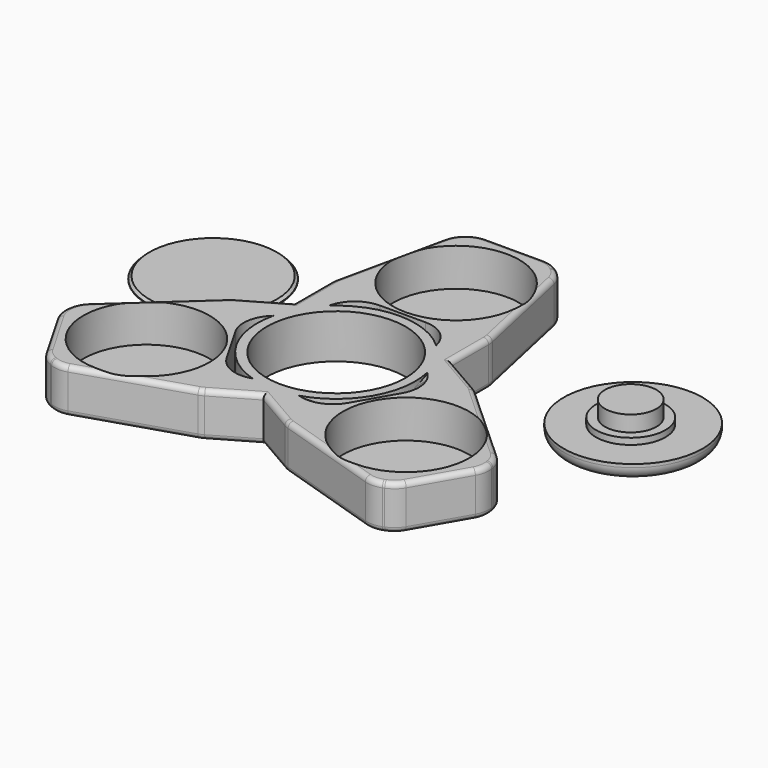
from build123d import *

# Parameters (mm, degrees)
F0_R         = 11
F1_DEPTH     = 7
F0_R_2       = 10
F2_DEPTH     = 7
F3_DEPTH     = 1
F4_SIZE      = 2
F5_R         = 4
F6_T3_DEPTH  = 17.2209539542
F6_T6_ANGLE  = 38.8320169601
F6_T9_ANGLE  = 38.8320169601
F6_T12_DEPTH = 9.1802464008
F6_T15_DEPTH = 0.2962051646
F6_T18_ANGLE = 38.8319208499
F6_T21_ANGLE = 38.8319208499
F6_T24_DEPTH = 17.2206278221
F6_T27_ANGLE = 12.3359660798
F6_T30_ANGLE = 38.8320169601
F6_T33_ANGLE = 38.8320169601
F6_T36_DEPTH = 17.2209539542
F6_T39_DEPTH = 9.1802464008
F6_T42_ANGLE = 38.8319208499
F6_T45_ANGLE = 38.8319208499
F6_T48_DEPTH = 17.2206278221
F6_T51_DEPTH = 0.2962051646
F6_T54_DEPTH = 0.2961934139
F6_T57_ANGLE = 12.3361583003
F6_T60_ANGLE = 12.3359660798
F6_T63_DEPTH = 0.2961934139
F6_T66_ANGLE = 12.3361583003
F6_T69_DEPTH = 14.5444922906
F6_S70_R     = 12.5
F6_T71_DEPTH = 9
F6_T74_DEPTH = 14.5441683265
F6_S75_R     = 12.5
F6_T76_DEPTH = 9
F6_T79_DEPTH = 14.5444922906
F6_S80_R     = 12.5
F6_T81_DEPTH = 9
F6_T84_DEPTH = 14.5441683265
F6_S85_R     = 12.5
F6_T86_DEPTH = 9
F7_T1_DEPTH  = 7
F8_COUNT     = 3
F9_R         = 10.5
F10_DEPTH    = 0.5
F11_SIZE     = 0.4
F12_R        = 11
F12_R_2      = 5.5
F13_DEPTH    = 2.5
F12_R_3      = 4.075
F14_DEPTH    = 3.5
F15_DEPTH    = 6
F16_R        = 2


# Not quite as in the source:
# - a fillet or chamfer that OpenCascade refuses, or shapes differently, is made with other operations: its cross-section is extruded or revolved along the edge and cut away or added


with BuildPart() as f1:
    # F0 (on Top) → F1 (new body)
    with BuildSketch(Plane.XY):
        with BuildLine():
            ThreePointArc((-12.5, 0), (0, -12.5), (12.5, 0))
            ThreePointArc((12.5, 0), (11.4564392374, 5), (8.5, 9.1651513899))
            ThreePointArc((8.5, 9.1651513899), (0, 12.5), (-8.5, 9.1651513899))
            ThreePointArc((-8.5, 9.1651513899), (-11.4564392374, 5), (-12.5, 0))
        make_face()
        Circle(F0_R, mode=Mode.SUBTRACT)
    extrude(amount=F1_DEPTH)

    # F0 (on Top) → F2 (join)
    with BuildSketch(Plane.XY):
        with BuildLine():
            ThreePointArc((8.5, 9.1651513899), (11.4564392374, 5), (12.5, 0))
            Line((12.5, 0), (12.5, 14.9764459367))
            Line((12.5, 14.9764459367), (8, 35.553243875))
            Line((8, 35.553243875), (0, 35.553243875))
            Line((0, 35.553243875), (-8, 35.553243875))
            Line((-8, 35.553243875), (-12.5, 14.9767766889))
            Line((-12.5, 14.9767766889), (-12.5, 0))
            ThreePointArc((-12.5, 0), (-11.4564392374, 5), (-8.5, 9.1651513899))
            Line((-8.5, 9.1651513899), (-8.5, 13.1651513899))
            Line((-8.5, 13.1651513899), (8.5, 13.1651513899))
            Line((8.5, 13.1651513899), (8.5, 9.1651513899))
        make_face()
        with Locations((0, 23.7397756428)):
            Circle(F0_R_2, mode=Mode.SUBTRACT)
    extrude(amount=F2_DEPTH)

    # F0 (on Top) → F3 (join)
    with BuildSketch(Plane.XY):
        with Locations((0, 23.7397756428)):
            Circle(F0_R_2)
    extrude(amount=F3_DEPTH)

    # F4
    f4_edges = [f1.edges().sort_by_distance(p)[0] for p in [
        (8, 35.553244, 3.5),
        (-8, 35.553244, 3.5),
    ]]
    chamfer(f4_edges, length=F4_SIZE)

    # F5
    f5_edges = [f1.edges().sort_by_distance(p)[0] for p in [
        (8.427287, 33.599421, 3.5),
        (6, 35.553244, 3.5),
        (-6, 35.553244, 3.5),
        (-8.427294, 33.599422, 3.5),
        (-12.5, 14.976777, 3.5),
        (12.5, 14.976446, 3.5),
    ]]
    fillet(f5_edges, radius=F5_R)

    # F6: fillet of radius 0.8 on 22 edges, made by hand


with BuildPart() as f6_tool1:
    # F6_s2 → F6_t3 (new body)
    with BuildSketch(Plane(origin=(-2.647556956, 12.1062765587, 0), x_dir=(0, 0, 1), z_dir=(-0.2136436617, 0.9769116571, 0))):
        with BuildLine():
            ThreePointArc((7, 14.6110184628), (6.7656854249, 15.1767038878), (6.2, 15.4110184628))
            Line((6.2, 15.4110184628), (7, 15.4110184628))
            Line((7, 15.4110184628), (7, 14.6110184628))
        make_face()
    extrude(amount=F6_T3_DEPTH)


with BuildPart() as f6_tool4:
    # F6_s5 → F6_t6 (revolve)
    with BuildSketch(Plane(origin=(-6.3267046163, 28.9296272233, 0), x_dir=(0, 0, 1), z_dir=(0.2136436617, -0.9769116571, 0))):
        with BuildLine():
            ThreePointArc((7, -14.6110184628), (6.7656854249, -15.1767038878), (6.2, -15.4110184628))
            Line((6.2, -15.4110184628), (7, -15.4110184628))
            Line((7, -15.4110184628), (7, -14.6110184628))
        make_face()
    revolve(axis=Axis((4.8208523397, 31.3675189911, 7), (0, 0, 1)), revolution_arc=F6_T6_ANGLE)


with BuildPart() as f6_tool7:
    # F6_s8 → F6_t9 (revolve)
    with BuildSketch(Plane(origin=(-12.6269800609, 10.163975148, 0), x_dir=(0, 0, 1), z_dir=(0.7789876962, -0.6270392086, 0))):
        with BuildLine():
            ThreePointArc((7, -30.6577747906), (6.7656854249, -31.2234602155), (6.2, -31.4577747906))
            Line((6.2, -31.4577747906), (7, -31.4577747906))
            Line((7, -31.4577747906), (7, -30.6577747906))
        make_face()
    revolve(axis=Axis((4.5901213146, 31.553243875, 7), (0, 0, 1)), revolution_arc=F6_T9_ANGLE)


with BuildPart() as f6_tool10:
    # F6_s11 → F6_t12 (new body)
    with BuildSketch(Plane.YZ.offset(-4.5901250862)):
        with BuildLine():
            ThreePointArc((34.753243875, 7), (35.3189293, 6.7656854249), (35.553243875, 6.2))
            Line((35.553243875, 6.2), (35.553243875, 7))
            Line((35.553243875, 7), (34.753243875, 7))
        make_face()
    extrude(amount=F6_T12_DEPTH)


with BuildPart() as f6_tool13:
    # F6_s14 → F6_t15 (new body)
    with BuildSketch(Plane(origin=(12.6269589424, 10.1639232441, 0), x_dir=(0, 0, 1), z_dir=(-0.778988748, -0.6270379019, 0))):
        with BuildLine():
            ThreePointArc((7, 30.6578043459), (6.7656854249, 31.2234897709), (6.2, 31.4578043459))
            Line((6.2, 31.4578043459), (7, 31.4578043459))
            Line((7, 31.4578043459), (7, 30.6578043459))
        make_face()
    extrude(amount=F6_T15_DEPTH)


with BuildPart() as f6_tool16:
    # F6_s17 → F6_t18 (revolve)
    with BuildSketch(Plane.YZ.offset(-4.5901250862)):
        with BuildLine():
            ThreePointArc((34.753243875, 7), (35.3189293, 6.7656854249), (35.553243875, 6.2))
            Line((35.553243875, 6.2), (35.553243875, 7))
            Line((35.553243875, 7), (34.753243875, 7))
        make_face()
    revolve(axis=Axis((-4.5901250862, 31.553243875, 7), (0, 0, 1)), revolution_arc=F6_T18_ANGLE)


with BuildPart() as f6_tool19:
    # F6_s20 → F6_t21 (revolve)
    with BuildSketch(Plane(origin=(12.3962184521, 9.9781913792, 0), x_dir=(0, 0, 1), z_dir=(0.778988748, 0.6270379019, 0))):
        with BuildLine():
            ThreePointArc((7, -30.6578043459), (6.7656854249, -31.2234897709), (6.2, -31.4578043459))
            Line((6.2, -31.4578043459), (7, -31.4578043459))
            Line((7, -31.4578043459), (7, -30.6578043459))
        make_face()
    revolve(axis=Axis((-4.8208655765, 31.3675120101, 7), (0, 0, 1)), revolution_arc=F6_T21_ANGLE)


with BuildPart() as f6_tool22:
    # F6_s23 → F6_t24 (new body)
    with BuildSketch(Plane(origin=(6.3267914314, 28.9295591739, 0), x_dir=(0, 0, 1), z_dir=(-0.2136469391, -0.9769109404, 0))):
        with BuildLine():
            ThreePointArc((7, 14.6111292517), (6.7656854249, 15.1768146767), (6.2, 15.4111292517))
            Line((6.2, 15.4111292517), (7, 15.4111292517))
            Line((7, 15.4111292517), (7, 14.6111292517))
        make_face()
    extrude(amount=F6_T24_DEPTH)


with BuildPart() as f6_tool25:
    # F6_s26 → F6_t27 (revolve)
    with BuildSketch(Plane(origin=(-2.647556956, 12.1062765587, 0), x_dir=(0, 0, 1), z_dir=(-0.2136436617, 0.9769116571, 0))):
        with BuildLine():
            ThreePointArc((7, 14.6110184628), (6.7656854249, 15.1767038878), (6.2, 15.4110184628))
            Line((6.2, 15.4110184628), (7, 15.4110184628))
            Line((7, 15.4110184628), (7, 14.6110184628))
        make_face()
    revolve(axis=Axis((8.5, 14.5441683265, 7), (0, 0, -1)), revolution_arc=F6_T27_ANGLE)


with BuildPart() as f6_tool28:
    # F6_s29 → F6_t30 (revolve)
    with BuildSketch(Plane(origin=(-12.6269800609, 10.163975148, 0), x_dir=(0, 0, 1), z_dir=(0.7789876962, -0.6270392086, 0))):
        with BuildLine():
            ThreePointArc((0.8, -31.4577747906), (0.2343145751, -31.2234602155), (0, -30.6577747906))
            Line((0, -30.6577747906), (0, -31.4577747906))
            Line((0, -31.4577747906), (0.8, -31.4577747906))
        make_face()
    revolve(axis=Axis((4.5901213146, 31.553243875, 0), (0, 0, 1)), revolution_arc=F6_T30_ANGLE)


with BuildPart() as f6_tool31:
    # F6_s32 → F6_t33 (revolve)
    with BuildSketch(Plane(origin=(-6.3267046163, 28.9296272233, 0), x_dir=(0, 0, 1), z_dir=(0.2136436617, -0.9769116571, 0))):
        with BuildLine():
            ThreePointArc((0.8, -15.4110184628), (0.2343145751, -15.1767038878), (0, -14.6110184628))
            Line((0, -14.6110184628), (0, -15.4110184628))
            Line((0, -15.4110184628), (0.8, -15.4110184628))
        make_face()
    revolve(axis=Axis((4.8208523397, 31.3675189911, 0), (0, 0, 1)), revolution_arc=F6_T33_ANGLE)


with BuildPart() as f6_tool34:
    # F6_s35 → F6_t36 (new body)
    with BuildSketch(Plane(origin=(-2.647556956, 12.1062765587, 0), x_dir=(0, 0, 1), z_dir=(-0.2136436617, 0.9769116571, 0))):
        with BuildLine():
            ThreePointArc((0.8, 15.4110184628), (0.2343145751, 15.1767038878), (0, 14.6110184628))
            Line((0, 14.6110184628), (0, 15.4110184628))
            Line((0, 15.4110184628), (0.8, 15.4110184628))
        make_face()
    extrude(amount=F6_T36_DEPTH)


with BuildPart() as f6_tool37:
    # F6_s38 → F6_t39 (new body)
    with BuildSketch(Plane.YZ.offset(4.5901213146)):
        with BuildLine():
            ThreePointArc((35.553243875, 0.8), (35.3189293, 0.2343145751), (34.753243875, 0))
            Line((34.753243875, 0), (35.553243875, 0))
            Line((35.553243875, 0), (35.553243875, 0.8))
        make_face()
    extrude(amount=-F6_T39_DEPTH)


with BuildPart() as f6_tool40:
    # F6_s41 → F6_t42 (revolve)
    with BuildSketch(Plane.YZ.offset(-4.5901250862)):
        with BuildLine():
            ThreePointArc((35.553243875, 0.8), (35.3189293, 0.2343145751), (34.753243875, 0))
            Line((34.753243875, 0), (35.553243875, 0))
            Line((35.553243875, 0), (35.553243875, 0.8))
        make_face()
    revolve(axis=Axis((-4.5901250862, 31.553243875, 0), (0, 0, 1)), revolution_arc=F6_T42_ANGLE)


with BuildPart() as f6_tool43:
    # F6_s44 → F6_t45 (revolve)
    with BuildSketch(Plane(origin=(12.3962184521, 9.9781913792, 0), x_dir=(0, 0, 1), z_dir=(0.778988748, 0.6270379019, 0))):
        with BuildLine():
            ThreePointArc((0.8, -31.4578043459), (0.2343145751, -31.2234897709), (0, -30.6578043459))
            Line((0, -30.6578043459), (0, -31.4578043459))
            Line((0, -31.4578043459), (0.8, -31.4578043459))
        make_face()
    revolve(axis=Axis((-4.8208655765, 31.3675120101, 0), (0, 0, 1)), revolution_arc=F6_T45_ANGLE)


with BuildPart() as f6_tool46:
    # F6_s47 → F6_t48 (new body)
    with BuildSketch(Plane(origin=(6.3267914314, 28.9295591739, 0), x_dir=(0, 0, 1), z_dir=(-0.2136469391, -0.9769109404, 0))):
        with BuildLine():
            ThreePointArc((0.8, 15.4111292517), (0.2343145751, 15.1768146767), (0, 14.6111292517))
            Line((0, 14.6111292517), (0, 15.4111292517))
            Line((0, 15.4111292517), (0.8, 15.4111292517))
        make_face()
    extrude(amount=F6_T48_DEPTH)


with BuildPart() as f6_tool49:
    # F6_s50 → F6_t51 (new body)
    with BuildSketch(Plane(origin=(12.6269589424, 10.1639232441, 0), x_dir=(0, 0, 1), z_dir=(-0.778988748, -0.6270379019, 0))):
        with BuildLine():
            ThreePointArc((0.8, 31.4578043459), (0.2343145751, 31.2234897709), (0, 30.6578043459))
            Line((0, 30.6578043459), (0, 31.4578043459))
            Line((0, 31.4578043459), (0.8, 31.4578043459))
        make_face()
    extrude(amount=F6_T51_DEPTH)


with BuildPart() as f6_tool52:
    # F6_s53 → F6_t54 (new body)
    with BuildSketch(Plane(origin=(-12.3962490358, 9.9782502642, 0), x_dir=(0, 0, 1), z_dir=(-0.7789876962, 0.6270392086, 0))):
        with BuildLine():
            ThreePointArc((7, 30.6577747906), (6.7656854249, 31.2234602155), (6.2, 31.4577747906))
            Line((6.2, 31.4577747906), (7, 31.4577747906))
            Line((7, 31.4577747906), (7, 30.6577747906))
        make_face()
    extrude(amount=F6_T54_DEPTH)


with BuildPart() as f6_tool55:
    # F6_s56 → F6_t57 (revolve)
    with BuildSketch(Plane.XZ.offset(-14.5444922906)):
        with BuildLine():
            ThreePointArc((-11.7, 7), (-12.2656854249, 6.7656854249), (-12.5, 6.2))
            Line((-12.5, 6.2), (-12.5, 7))
            Line((-12.5, 7), (-11.7, 7))
        make_face()
    revolve(axis=Axis((-8.5, 14.5444922906, 7), (0, 0, -1)), revolution_arc=F6_T57_ANGLE)


with BuildPart() as f6_tool58:
    # F6_s59 → F6_t60 (revolve)
    with BuildSketch(Plane(origin=(-2.647556956, 12.1062765587, 0), x_dir=(0, 0, 1), z_dir=(-0.2136436617, 0.9769116571, 0))):
        with BuildLine():
            ThreePointArc((0.8, 15.4110184628), (0.2343145751, 15.1767038878), (0, 14.6110184628))
            Line((0, 14.6110184628), (0, 15.4110184628))
            Line((0, 15.4110184628), (0.8, 15.4110184628))
        make_face()
    revolve(axis=Axis((8.5, 14.5441683265, 0), (0, 0, -1)), revolution_arc=F6_T60_ANGLE)


with BuildPart() as f6_tool61:
    # F6_s62 → F6_t63 (new body)
    with BuildSketch(Plane(origin=(-12.3962490358, 9.9782502642, 0), x_dir=(0, 0, 1), z_dir=(-0.7789876962, 0.6270392086, 0))):
        with BuildLine():
            ThreePointArc((0.8, 31.4577747906), (0.2343145751, 31.2234602155), (0, 30.6577747906))
            Line((0, 30.6577747906), (0, 31.4577747906))
            Line((0, 31.4577747906), (0.8, 31.4577747906))
        make_face()
    extrude(amount=F6_T63_DEPTH)


with BuildPart() as f6_tool64:
    # F6_s65 → F6_t66 (revolve)
    with BuildSketch(Plane.XZ.offset(-14.5444922906)):
        with BuildLine():
            ThreePointArc((-12.5, 0.8), (-12.2656854249, 0.2343145751), (-11.7, 0))
            Line((-11.7, 0), (-12.5, 0))
            Line((-12.5, 0), (-12.5, 0.8))
        make_face()
    revolve(axis=Axis((-8.5, 14.5444922906, 0), (0, 0, -1)), revolution_arc=F6_T66_ANGLE)


with BuildPart() as f6_tool67:
    # F6_s68 → F6_t69 (new body)
    with BuildSketch(Plane.XZ.offset(-14.5444922906)):
        with BuildLine():
            ThreePointArc((-12.5, 0.8), (-12.2656854249, 0.2343145751), (-11.7, 0))
            Line((-11.7, 0), (-12.5, 0))
            Line((-12.5, 0), (-12.5, 0.8))
        make_face()
    extrude(amount=F6_T69_DEPTH)

    # F6_s70 → F6_t71 (cut, symmetric)
    with BuildSketch(Plane.XY.offset(0.4)):
        Circle(F6_S70_R)
    extrude(amount=F6_T71_DEPTH, both=True, mode=Mode.SUBTRACT)


with BuildPart() as f6_tool72:
    # F6_s73 → F6_t74 (new body)
    with BuildSketch(Plane.XZ):
        with BuildLine():
            ThreePointArc((12.5, 0.8), (12.2656854249, 0.2343145751), (11.7, 0))
            Line((11.7, 0), (12.5, 0))
            Line((12.5, 0), (12.5, 0.8))
        make_face()
    extrude(amount=-F6_T74_DEPTH)

    # F6_s75 → F6_t76 (cut, symmetric)
    with BuildSketch(Plane.XY.offset(0.4)):
        Circle(F6_S75_R)
    extrude(amount=F6_T76_DEPTH, both=True, mode=Mode.SUBTRACT)


with BuildPart() as f6_tool77:
    # F6_s78 → F6_t79 (new body)
    with BuildSketch(Plane.XZ.offset(-14.5444922906)):
        with BuildLine():
            ThreePointArc((-11.7, 7), (-12.2656854249, 6.7656854249), (-12.5, 6.2))
            Line((-12.5, 6.2), (-12.5, 7))
            Line((-12.5, 7), (-11.7, 7))
        make_face()
    extrude(amount=F6_T79_DEPTH)

    # F6_s80 → F6_t81 (cut, symmetric)
    with BuildSketch(Plane.XY.offset(6.6)):
        Circle(F6_S80_R)
    extrude(amount=F6_T81_DEPTH, both=True, mode=Mode.SUBTRACT)


with BuildPart() as f6_tool82:
    # F6_s83 → F6_t84 (new body)
    with BuildSketch(Plane.XZ):
        with BuildLine():
            ThreePointArc((11.7, 7), (12.2656854249, 6.7656854249), (12.5, 6.2))
            Line((12.5, 6.2), (12.5, 7))
            Line((12.5, 7), (11.7, 7))
        make_face()
    extrude(amount=-F6_T84_DEPTH)

    # F6_s85 → F6_t86 (cut, symmetric)
    with BuildSketch(Plane.XY.offset(6.6)):
        Circle(F6_S85_R)
    extrude(amount=F6_T86_DEPTH, both=True, mode=Mode.SUBTRACT)


with BuildPart() as f1_1:
    add(f1.part)

    # F6_t87: cut F6_tool1, F6_tool4, F6_tool7, F6_tool10, F6_tool13, F6_tool16, F6_tool19, F6_tool22, F6_tool25, F6_tool28, F6_tool31, F6_tool34, F6_tool37, F6_tool40, F6_tool43, F6_tool46, F6_tool49, F6_tool52, F6_tool55, F6_tool58, F6_tool61, F6_tool64, F6_tool67, F6_tool72, F6_tool77, F6_tool82
    add([f6_tool1.part, f6_tool4.part, f6_tool7.part, f6_tool10.part, f6_tool13.part, f6_tool16.part, f6_tool19.part, f6_tool22.part, f6_tool25.part, f6_tool28.part, f6_tool31.part, f6_tool34.part, f6_tool37.part, f6_tool40.part, f6_tool43.part, f6_tool46.part, f6_tool49.part, f6_tool52.part, f6_tool55.part, f6_tool58.part, f6_tool61.part, f6_tool64.part, f6_tool67.part, f6_tool72.part, f6_tool77.part, f6_tool82.part], mode=Mode.SUBTRACT)

    # F7: fillet of radius 5 on 2 edges, made by hand

    # F7_s2 → F7_t1 (join)
    with BuildSketch(Plane.XY):
        with BuildLine():
            ThreePointArc((-8.5, 9.1651513899), (-6.7632981746, 12.0381347361), (-3.6010205144, 13.1651513899))
            Line((-3.6010205144, 13.1651513899), (-8.5, 13.1651513899))
            Line((-8.5, 13.1651513899), (-8.5, 9.1651513899))
        make_face()
        with BuildLine():
            ThreePointArc((8.5, 9.1651513899), (6.7632981746, 12.0381347361), (3.6010205144, 13.1651513899))
            Line((3.6010205144, 13.1651513899), (8.5, 13.1651513899))
            Line((8.5, 13.1651513899), (8.5, 9.1651513899))
        make_face()
    extrude(amount=F7_T1_DEPTH)

    # F8: F1 ×3 about axis
    f8_axis = Axis((0, 0, 7), (0, 0, 1))


with BuildPart() as f1_2:
    add(f1_1.part)
    for i in range(1, F8_COUNT):
        add(f1_1.part.rotate(f8_axis, i * 360 / F8_COUNT))


with BuildPart() as f10:
    # F9 (on Top) → F10 (new body)
    with BuildSketch(Plane.XY):
        with Locations((-32.494250685, 16.2477288395)):
            Circle(F9_R)
    extrude(amount=F10_DEPTH)

    # F11
    f11_edges = [f10.edges().sort_by_distance(p)[0] for p in [
        (-42.994251, 16.247729, 0.5),
    ]]
    chamfer(f11_edges, length=F11_SIZE)


with BuildPart() as f13:
    # F12 (on Top) → F13 (new body)
    with BuildSketch(Plane.XY):
        with Locations((35.1202301681, 14.8915722966)):
            Circle(F12_R)
        with Locations((35.1202301681, 14.4120967016)):
            Circle(F12_R_2, mode=Mode.SUBTRACT)
    extrude(amount=F13_DEPTH)

    # F12 (on Top) → F14 (join)
    with BuildSketch(Plane.XY):
        with Locations((35.1202301681, 14.4120967016)):
            Circle(F12_R_2)
        with Locations((35.1202301681, 14.4120967016)):
            Circle(F12_R_3, mode=Mode.SUBTRACT)
    extrude(amount=F14_DEPTH)

    # F12 (on Top) → F15 (join)
    with BuildSketch(Plane.XY):
        with Locations((35.1202301681, 14.4120967016)):
            Circle(F12_R_3)
    extrude(amount=F15_DEPTH)

    # F16
    f16_edges = [f13.edges().sort_by_distance(p)[0] for p in [
        (24.12023, 14.891572, 0),
    ]]
    fillet(f16_edges, radius=F16_R)


solid = Compound([f1_2.part, f10.part, f13.part])
